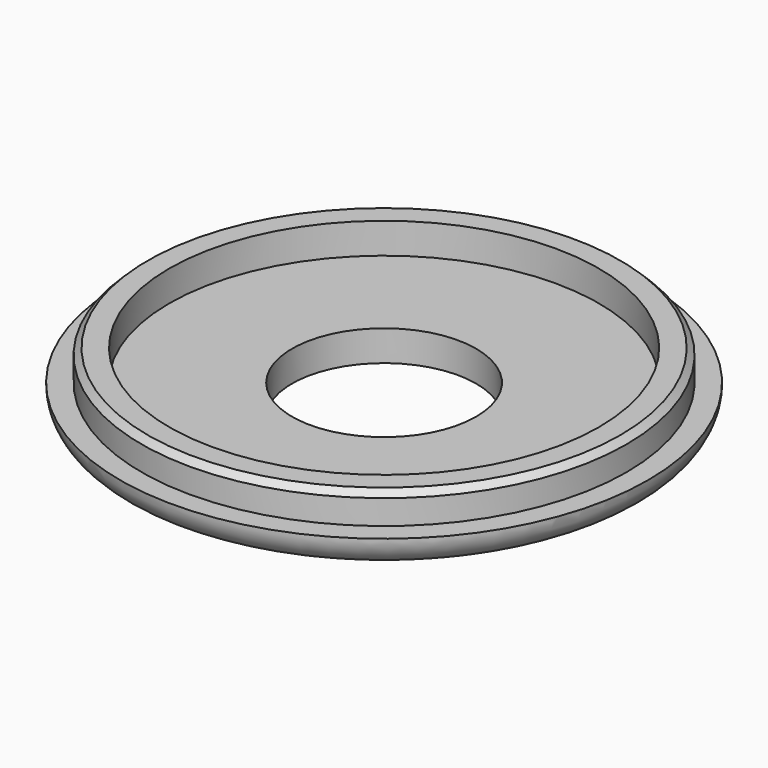
from build123d import *

# Parameters (mm, degrees)
F0_R     = 39.5
F0_R_2   = 35
F1_DEPTH = 5
F0_R_3   = 43
F0_R_4   = 15
F2_DEPTH = 5
F3_R     = 4.99999
F4_SIZE  = 1


# Not quite as in the source:
# - a fillet or chamfer is up to 0.001 mm smaller than in the source, because OpenCascade refuses the exact size


with BuildPart() as f1:
    # F0 (on Top) → F1 (new body)
    with BuildSketch(Plane.XY):
        Circle(F0_R)
        Circle(F0_R_2, mode=Mode.SUBTRACT)
    extrude(amount=F1_DEPTH)

    # F0 (on Top) → F2 (join)
    with BuildSketch(Plane.XY):
        Circle(F0_R_3)
        Circle(F0_R, mode=Mode.SUBTRACT)
        Circle(F0_R)
        Circle(F0_R_2, mode=Mode.SUBTRACT)
        Circle(F0_R_2)
        Circle(F0_R_4, mode=Mode.SUBTRACT)
    extrude(amount=-F2_DEPTH)

    # F3 (radius 5 in the source; OpenCascade refuses exactly that, so slightly less here)
    f3_edges = [f1.edges().sort_by_distance(p)[0] for p in [
        (-43, 0, -5),
    ]]
    fillet(f3_edges, radius=F3_R)

    # F4
    f4_edges = [f1.edges().sort_by_distance(p)[0] for p in [
        (-39.5, 0, 5),
    ]]
    chamfer(f4_edges, length=F4_SIZE)


solid = f1.part
